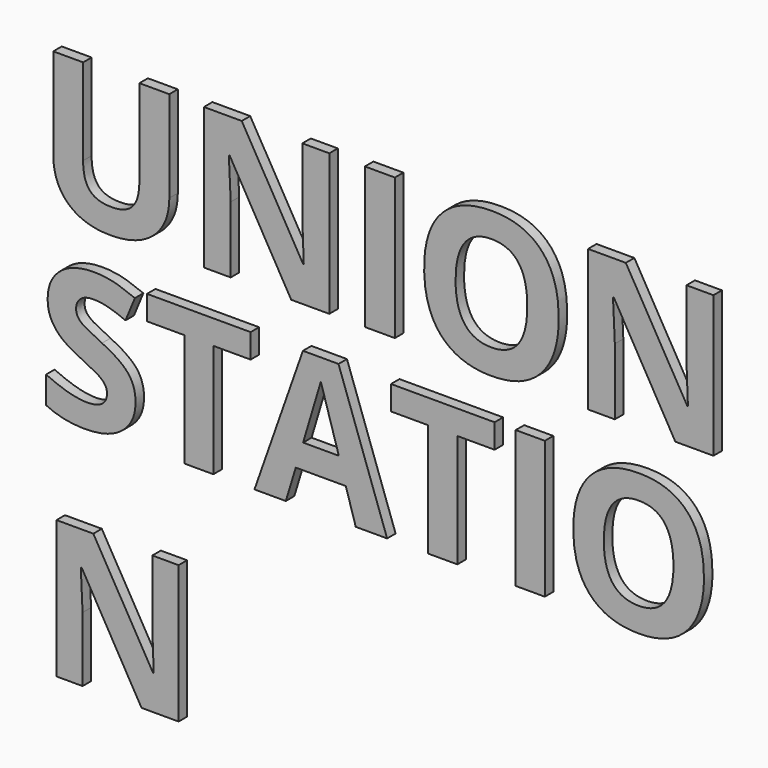
from build123d import *

# Parameters (mm, degrees)
F0_TEXT_SIZE   = 710.8981410662
F1_DEPTH       = 38.1
F0_TEXT_SIZE_2 = 690.2454774647
F2_DEPTH       = 38.1
F0_TEXT_SIZE_3 = 692.3908988635
F3_DEPTH       = 38.1


# Not quite as in the source:
# - Text() gives the source's letters only with a copy of the font that has no kerning and outlines rounded to 1/6400 em; it was checked with that copy


with BuildPart() as f1:
    # F0 (on Front) → F1 (new body)
    with BuildSketch(Plane.XZ):
        with Locations((-1219.2, -246.1187541485)):
            Text('UNION', F0_TEXT_SIZE, font='Open Sans', font_style=FontStyle.BOLD, text_align=(TextAlign.LEFT, TextAlign.BOTTOM))
    extrude(amount=F1_DEPTH)


with BuildPart() as f2:
    # F0 (on Front) → F2 (new body)
    with BuildSketch(Plane.XZ):
        with Locations((-1216.2885665894, -888.4296651141)):
            Text('STATIO', F0_TEXT_SIZE_2, font='Open Sans', font_style=FontStyle.BOLD, text_align=(TextAlign.LEFT, TextAlign.BOTTOM))
    extrude(amount=F2_DEPTH)


with BuildPart() as f3:
    # F0 (on Front) → F3 (new body)
    with BuildSketch(Plane.XZ):
        with Locations((-1209.4480991364, -1710.6561660767)):
            Text('N', F0_TEXT_SIZE_3, font='Open Sans', font_style=FontStyle.BOLD, text_align=(TextAlign.LEFT, TextAlign.BOTTOM))
    extrude(amount=F3_DEPTH)


solid = Compound([f1.part, f2.part, f3.part])
